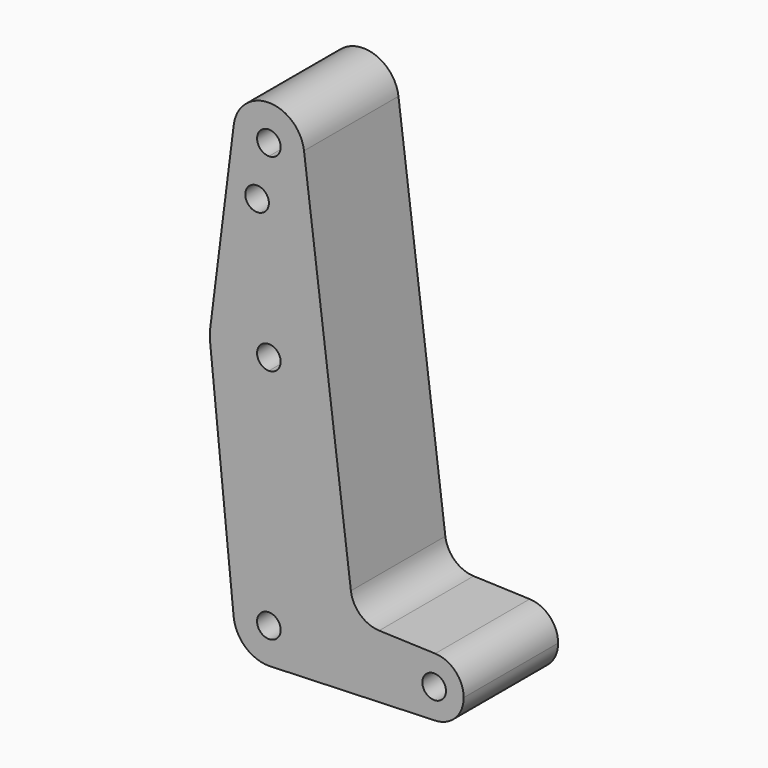
from build123d import *

# Parameters (mm, degrees)
F0_R     = 3.175
F1_DEPTH = 31.75


with BuildPart() as f1:
    # F0 (on Front) → F1 (new body)
    with BuildSketch(Plane.XZ):
        with BuildLine():
            Line((22.0577025061, 15.4224140263), (15.7504882737, 65.484375))
            ThreePointArc((15.7504882737, 65.484375), (15.8438414904, 64.4941387366), (15.875, 63.5))
            ThreePointArc((15.875, 63.5), (11.2253201513, 52.2746798487), (0, 47.625))
            Line((0, 47.625), (0, 9.525))
            ThreePointArc((0, 9.525), (6.7351920908, 6.7351920908), (9.525, 0))
            Line((9.525, 0), (36.5125, 0))
            ThreePointArc((36.5125, 0), (38.9384772185, 5.7120069047), (44.7334821429, 7.9324362036))
            Line((44.7334821429, 7.9324362036), (29.6616113193, 8.4710609247))
            ThreePointArc((29.6616113193, 8.4710609247), (24.5813298898, 10.5484079743), (22.0577025061, 15.4224140263))
        make_face()
        with BuildLine():
            ThreePointArc((9.4502929642, 115.490625), (9.5063048942, 114.896483242), (9.525, 114.3))
            ThreePointArc((9.525, 114.3), (6.7351920908, 107.5648079092), (0, 104.775))
            Line((0, 104.775), (0, 100.0252))
            Line((0, 100.0252), (0, 79.375))
            ThreePointArc((0, 79.375), (10.5003255158, 75.40625), (15.7504882737, 65.484375))
            Line((15.7504882737, 65.484375), (9.4502929642, 115.490625))
        make_face()
        with BuildLine():
            Line((0, 100.0252), (0, 104.775))
            ThreePointArc((0, 104.775), (-7.14375, 107.9998046905), (-9.4502929642, 115.490625))
            Line((-9.4502929642, 115.490625), (-15.7504882737, 65.484375))
            ThreePointArc((-15.7504882737, 65.484375), (-10.5003255158, 75.40625), (0, 79.375))
            Line((0, 79.375), (0, 100.0252))
        make_face()
        with Locations((-3.175, 100.0252)):
            Circle(F0_R, mode=Mode.SUBTRACT)
        with BuildLine():
            ThreePointArc((0, 104.775), (6.7351920908, 107.5648079092), (9.525, 114.3))
            ThreePointArc((9.525, 114.3), (9.5063048942, 114.896483242), (9.4502929642, 115.490625))
            ThreePointArc((9.4502929642, 115.490625), (0, 123.825), (-9.4502929642, 115.490625))
            ThreePointArc((-9.4502929642, 115.490625), (-7.14375, 107.9998046905), (0, 104.775))
        make_face()
        with BuildLine():
            ThreePointArc((3.175, 114.3), (2.2450640303, 112.0549359697), (0, 111.125))
            ThreePointArc((0, 111.125), (-2.2450640303, 116.5450640303), (3.175, 114.3))
        make_face(mode=Mode.SUBTRACT)
        with BuildLine():
            Line((36.5125, 0), (9.525, 0))
            ThreePointArc((9.525, 0), (6.9705567315, -6.4912990883), (0.6773435479, -9.500885786))
            Line((0.6773435479, -9.500885786), (44.7324052746, -7.9324746146))
            ThreePointArc((44.7324052746, -7.9324746146), (38.9380895153, -5.7116327839), (36.5125, 0))
        make_face()
        with BuildLine():
            ThreePointArc((0, 9.525), (-7.063929059, 6.3895642457), (-9.4772553384, -0.9525))
            ThreePointArc((-9.4772553384, -0.9525), (-6.3895642457, -7.063929059), (0, -9.525))
            Line((0, -9.525), (0.6773435479, -9.500885786))
            ThreePointArc((0.6773435479, -9.500885786), (6.9705567315, -6.4912990883), (9.525, 0))
            Line((9.525, 0), (3.175, 0))
            ThreePointArc((3.175, 0), (-2.2450640303, -2.2450640303), (0, 3.175))
            Line((0, 3.175), (0, 9.525))
        make_face()
        with BuildLine():
            ThreePointArc((9.525, 0), (6.7351920908, 6.7351920908), (0, 9.525))
            Line((0, 9.525), (0, 3.175))
            ThreePointArc((0, 3.175), (2.2450640303, 2.2450640303), (3.175, 0))
            Line((3.175, 0), (9.525, 0))
        make_face()
        with BuildLine():
            ThreePointArc((52.3875, 0), (50.1620069047, 5.5115227815), (44.7334821429, 7.9324362036))
            ThreePointArc((44.7334821429, 7.9324362036), (38.9384772185, 5.7120069047), (36.5125, 0))
            ThreePointArc((36.5125, 0), (38.9380895153, -5.7116327839), (44.7324052746, -7.9324746146))
            ThreePointArc((44.7324052746, -7.9324746146), (50.1616327839, -5.5119104847), (52.3875, 0))
        make_face()
        with BuildLine():
            ThreePointArc((47.625, 0), (44.45, -3.175), (41.275, 0))
            ThreePointArc((41.275, 0), (44.45, 3.175), (47.625, 0))
        make_face(mode=Mode.SUBTRACT)
        with BuildLine():
            ThreePointArc((0, 79.375), (-10.5003255158, 75.40625), (-15.7504882737, 65.484375))
            ThreePointArc((-15.7504882737, 65.484375), (-15.8737438155, 63.6997054867), (-15.7954255641, 61.9125))
            ThreePointArc((-15.7954255641, 61.9125), (-10.6492737428, 51.7267849017), (0, 47.625))
            Line((0, 47.625), (0, 60.325))
            ThreePointArc((0, 60.325), (-3.175, 63.5), (0, 66.675))
            Line((0, 66.675), (0, 79.375))
        make_face()
        with BuildLine():
            ThreePointArc((15.875, 63.5), (15.8438414904, 64.4941387366), (15.7504882737, 65.484375))
            ThreePointArc((15.7504882737, 65.484375), (10.5003255158, 75.40625), (0, 79.375))
            Line((0, 79.375), (0, 66.675))
            ThreePointArc((0, 66.675), (2.2450640303, 65.7450640303), (3.175, 63.5))
            ThreePointArc((3.175, 63.5), (2.2450640303, 61.2549359697), (0, 60.325))
            Line((0, 60.325), (0, 47.625))
            ThreePointArc((0, 47.625), (11.2253201513, 52.2746798487), (15.875, 63.5))
        make_face()
        with BuildLine():
            ThreePointArc((0, 47.625), (-10.6492737428, 51.7267849017), (-15.7954255641, 61.9125))
            Line((-15.7954255641, 61.9125), (-9.4772553384, -0.9525))
            ThreePointArc((-9.4772553384, -0.9525), (-7.063929059, 6.3895642457), (0, 9.525))
            Line((0, 9.525), (0, 47.625))
        make_face()
    extrude(amount=F1_DEPTH)


solid = f1.part
